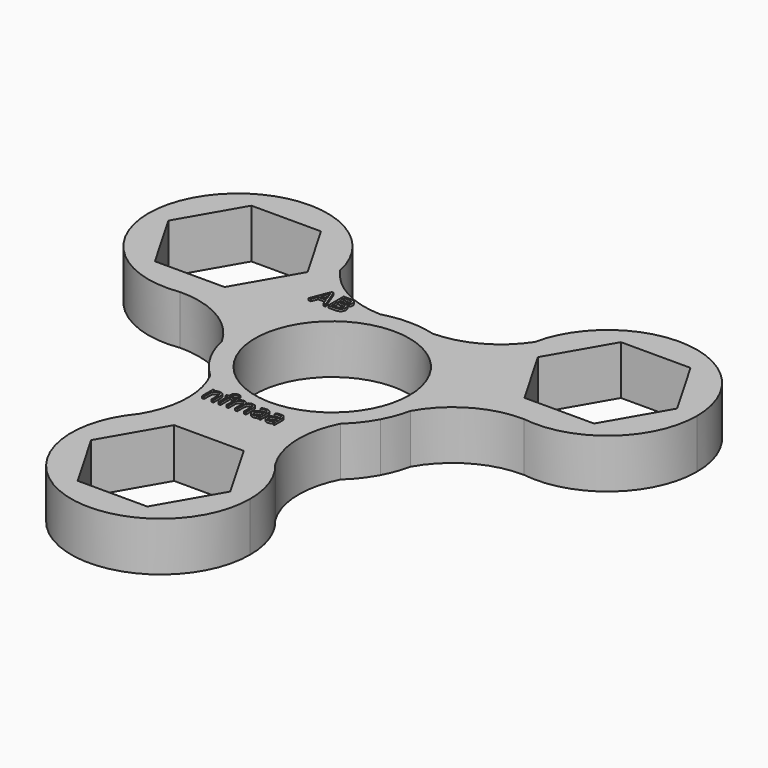
from build123d import *

# Parameters (mm, degrees)
F0_R           = 10.9873545291
F1_DEPTH       = 7
F2_TEXT_SIZE   = 3.6541450148
F2_TEXT_SIZE_2 = 3.8281509963
F3_DEPTH       = 7.3


# Not quite as in the source:
# - Text() gives the source's letters only with a copy of the font that has no kerning and outlines rounded to 1/6400 em; it was checked with that copy


with BuildPart() as f1:
    # F0 (on Top) → F1 (new body)
    with BuildSketch(Plane.XY):
        with BuildLine():
            ThreePointArc((13.4370735728, -2.8509917433), (13.6612112558, -1.4333203212), (13.7361967123, 0))
            ThreePointArc((13.7361967123, 0), (10.9474454774, 8.2967787508), (3.7135479281, 13.2246989344))
            ThreePointArc((3.7135479281, 13.2246989344), (1.8373418812, 13.3393680881), (0, 13.7361967123))
            ThreePointArc((0, 13.7361967123), (-1.8373418812, 13.3393680881), (-3.7135479281, 13.2246989344))
            ThreePointArc((-3.7135479281, 13.2246989344), (-11.7534212959, 7.1091622546), (-13.4370735728, -2.8509917433))
            ThreePointArc((-13.4370735728, -2.8509917433), (-12.6180956982, -4.6322934634), (-12.0899866465, -6.5203775204))
            ThreePointArc((-12.0899866465, -6.5203775204), (-10.5155940661, -8.1944331859), (-9.2770038263, -10.1301678232))
            ThreePointArc((-9.2770038263, -10.1301678232), (0, -13.7361967123), (9.2770038263, -10.1301678232))
            ThreePointArc((9.2770038263, -10.1301678232), (10.5155940661, -8.1944331859), (12.0899866465, -6.5203775204))
            ThreePointArc((12.0899866465, -6.5203775204), (12.6180956982, -4.6322934634), (13.4370735728, -2.8509917433))
        make_face()
        Circle(F0_R, mode=Mode.SUBTRACT)
        with BuildLine():
            ThreePointArc((3.7135479281, 13.2246989344), (10.9474454774, 8.2967787508), (13.7361967123, 0))
            ThreePointArc((13.7361967123, 0), (13.6612112558, -1.4333203212), (13.4370735728, -2.8509917433))
            ThreePointArc((13.4370735728, -2.8509917433), (18.0911751741, 1.8532858299), (24.5016416073, 3.4954823191))
            ThreePointArc((24.5016416073, 3.4954823191), (15.8734601267, 8.8049243257), (13.8399737887, 18.7296723525))
            ThreePointArc((13.8399737887, 18.7296723525), (9.4549244598, 14.7297003407), (3.7135479281, 13.2246989344))
        make_face()
        with BuildLine():
            ThreePointArc((0, 13.7361967123), (1.8373418812, 13.3393680881), (3.7135479281, 13.2246989344))
            ThreePointArc((3.7135479281, 13.2246989344), (1.874304417, 13.6077214504), (0, 13.7361967123))
        make_face()
        with BuildLine():
            ThreePointArc((12.0899866465, -6.5203775204), (12.8947198052, -4.7338463501), (13.4370735728, -2.8509917433))
            ThreePointArc((13.4370735728, -2.8509917433), (12.6180956982, -4.6322934634), (12.0899866465, -6.5203775204))
        make_face()
        with BuildLine():
            ThreePointArc((-3.7135479281, 13.2246989344), (-1.8373418812, 13.3393680881), (0, 13.7361967123))
            ThreePointArc((0, 13.7361967123), (-1.874304417, 13.6077214504), (-3.7135479281, 13.2246989344))
        make_face()
        with BuildLine():
            ThreePointArc((39.0710365567, 16.1160435528), (27.6339422462, 28.7990793083), (13.8399737887, 18.7296723525))
            ThreePointArc((13.8399737887, 18.7296723525), (15.8734601267, 8.8049243257), (24.5016416073, 3.4954823191))
            ThreePointArc((24.5016416073, 3.4954823191), (34.6687294807, 6.4782814286), (39.0710365567, 16.1160435528))
        make_face()
        Polygon((16.404276959, 16.1160435528), (21.3622060899, 24.7034287079), (31.2780643518, 24.7034287079), (36.2359934828, 16.1160435528), (31.2780643518, 7.5286583976), (21.3622060899, 7.5286583976), align=None, mode=Mode.SUBTRACT)
        with BuildLine():
            ThreePointArc((9.2770038263, -10.1301678232), (10.8348842621, -8.4432448233), (12.0899866465, -6.5203775204))
            ThreePointArc((12.0899866465, -6.5203775204), (10.5155940661, -8.1944331859), (9.2770038263, -10.1301678232))
        make_face()
        with BuildLine():
            ThreePointArc((-13.4370735728, -2.8509917433), (-11.7534212959, 7.1091622546), (-3.7135479281, 13.2246989344))
            ThreePointArc((-3.7135479281, 13.2246989344), (-9.4549244598, 14.7297003407), (-13.8399737887, 18.7296723525))
            ThreePointArc((-13.8399737887, 18.7296723525), (-13.6370994653, 17.429850578), (-13.5692338851, 16.1160435528))
            ThreePointArc((-13.5692338851, 16.1160435528), (-16.6823730968, 7.767449293), (-24.5016416073, 3.4954823191))
            ThreePointArc((-24.5016416073, 3.4954823191), (-18.0911751741, 1.8532858299), (-13.4370735728, -2.8509917433))
        make_face()
        with BuildLine():
            ThreePointArc((9.7041195554, -22.2696484463), (7.9030765909, -16.2557622423), (9.2770038263, -10.1301678232))
            ThreePointArc((9.2770038263, -10.1301678232), (0, -13.7361967123), (-9.2770038263, -10.1301678232))
            ThreePointArc((-9.2770038263, -10.1301678232), (-7.9030765909, -16.2557622423), (-9.7041195554, -22.2696484463))
            ThreePointArc((-9.7041195554, -22.2696484463), (0, -17.7901163157), (9.7041195554, -22.2696484463))
        make_face()
        with BuildLine():
            ThreePointArc((-12.0899866465, -6.5203775204), (-12.6180956982, -4.6322934634), (-13.4370735728, -2.8509917433))
            ThreePointArc((-13.4370735728, -2.8509917433), (-12.8947198052, -4.7338463501), (-12.0899866465, -6.5203775204))
        make_face()
        with BuildLine():
            ThreePointArc((-13.5692338851, 16.1160435528), (-13.6370994653, 17.429850578), (-13.8399737887, 18.7296723525))
            ThreePointArc((-13.8399737887, 18.7296723525), (-36.7668103151, 23.4271627798), (-24.5016416073, 3.4954823191))
            ThreePointArc((-24.5016416073, 3.4954823191), (-16.6823730968, 7.767449293), (-13.5692338851, 16.1160435528))
        make_face()
        Polygon((-31.2780643518, 7.5286583976), (-36.2359934828, 16.1160435528), (-31.2780643518, 24.7034287079), (-21.3622060899, 24.7034287079), (-16.404276959, 16.1160435528), (-21.3622060899, 7.5286583976), align=None, mode=Mode.SUBTRACT)
        with BuildLine():
            ThreePointArc((-12.0899866465, -6.5203775204), (-10.8348842621, -8.4432448233), (-9.2770038263, -10.1301678232))
            ThreePointArc((-9.2770038263, -10.1301678232), (-10.5155940661, -8.1944331859), (-12.0899866465, -6.5203775204))
        make_face()
        with BuildLine():
            ThreePointArc((12.7509013358, -30.5410176516), (11.9649854968, -26.133682069), (9.7041195554, -22.2696484463))
            ThreePointArc((9.7041195554, -22.2696484463), (0, -17.7901163157), (-9.7041195554, -22.2696484463))
            ThreePointArc((-9.7041195554, -22.2696484463), (-4.4073355825, -42.5060031484), (12.7509013358, -30.5410176516))
        make_face()
        Polygon((-9.9158582619, -30.5410176516), (-4.957929131, -21.9536324964), (4.957929131, -21.9536324964), (9.9158582619, -30.5410176516), (4.957929131, -39.1284028067), (-4.957929131, -39.1284028067), align=None, mode=Mode.SUBTRACT)
    extrude(amount=F1_DEPTH)

    # F2 (on Top) → F3 (join)
    with BuildSketch(Plane.XY):
        with Locations((-6.8894140422, -14.9661870673)):
            Text('nfmaa', F2_TEXT_SIZE, font='Open Sans', text_align=(TextAlign.LEFT, TextAlign.BOTTOM))
        with Locations((-12.0260966942, 10.8425142244)):
            Text('AB', F2_TEXT_SIZE_2, font='Open Sans', text_align=(TextAlign.LEFT, TextAlign.BOTTOM))
    extrude(amount=F3_DEPTH)


solid = f1.part
